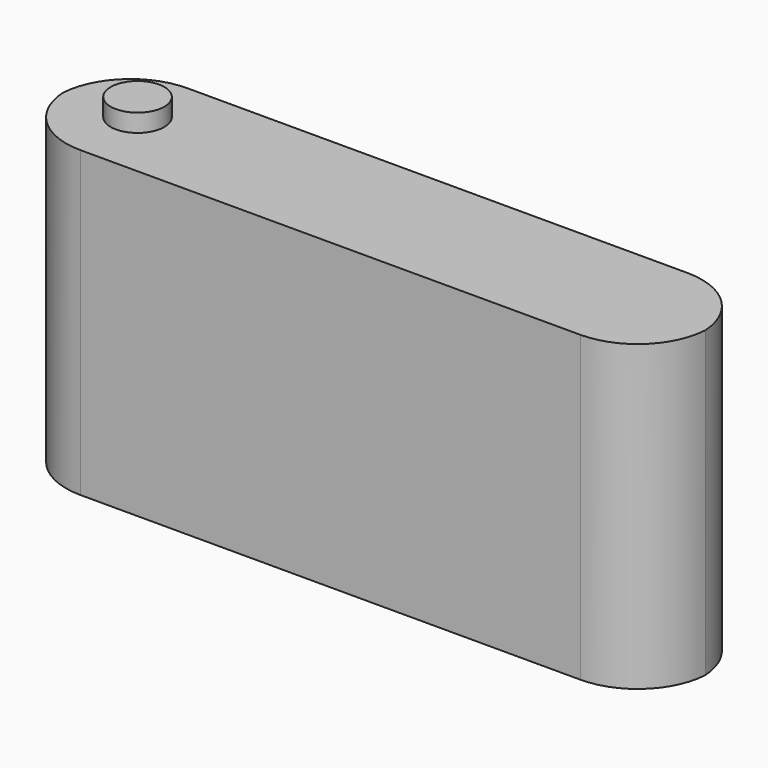
from build123d import *

# Parameters (mm, degrees)
F0_W        = 72
F0_H        = 34
F1_DEPTH    = 15
F2_T1_DEPTH = 74
F3_R        = 3
F4_DEPTH    = 2
F5_R        = 3
F6_DEPTH    = 2


# Not quite as in the source:
# - a fillet or chamfer that OpenCascade refuses, or shapes differently, is made with other operations: its cross-section is extruded or revolved along the edge and cut away or added


with BuildPart() as f1:
    # F0 (on Front) → F1 (new body)
    with BuildSketch(Plane.XZ):
        Rectangle(F0_W, F0_H)
    extrude(amount=F1_DEPTH)

    # F2: fillet of radius 8 on 4 edges, made by hand

    # F2_s2 → F2_t1 (cut)
    with BuildSketch(Plane.XY.offset(-37)):
        with BuildLine():
            ThreePointArc((-36, -8), (-33.6568542495, -2.3431457505), (-28, 0))
            Line((-28, 0), (-36, 0))
            Line((-36, 0), (-36, -8))
        make_face()
        with BuildLine():
            ThreePointArc((-36, -7), (-33.6568542495, -12.6568542495), (-28, -15))
            Line((-28, -15), (-36, -15))
            Line((-36, -15), (-36, -7))
        make_face()
        with BuildLine():
            ThreePointArc((36, -7), (33.6568542495, -12.6568542495), (28, -15))
            Line((28, -15), (36, -15))
            Line((36, -15), (36, -7))
        make_face()
        with BuildLine():
            ThreePointArc((36, -8), (33.6568542495, -2.3431457505), (28, 0))
            Line((28, 0), (36, 0))
            Line((36, 0), (36, -8))
        make_face()
    extrude(amount=F2_T1_DEPTH, mode=Mode.SUBTRACT)

    # F3 (on face) → F4 (join)
    with BuildSketch(Plane.XY.offset(17)):
        with Locations((-28, -7)):
            Circle(F3_R)
    extrude(amount=F4_DEPTH)

    # F5 (on face) → F6 (join)
    with BuildSketch(Plane(origin=(0, 0, -17), x_dir=(1, 0, 0), z_dir=(0, 0, -1))):
        with Locations((-28, 8)):
            Circle(F5_R)
    extrude(amount=F6_DEPTH)


solid = f1.part
